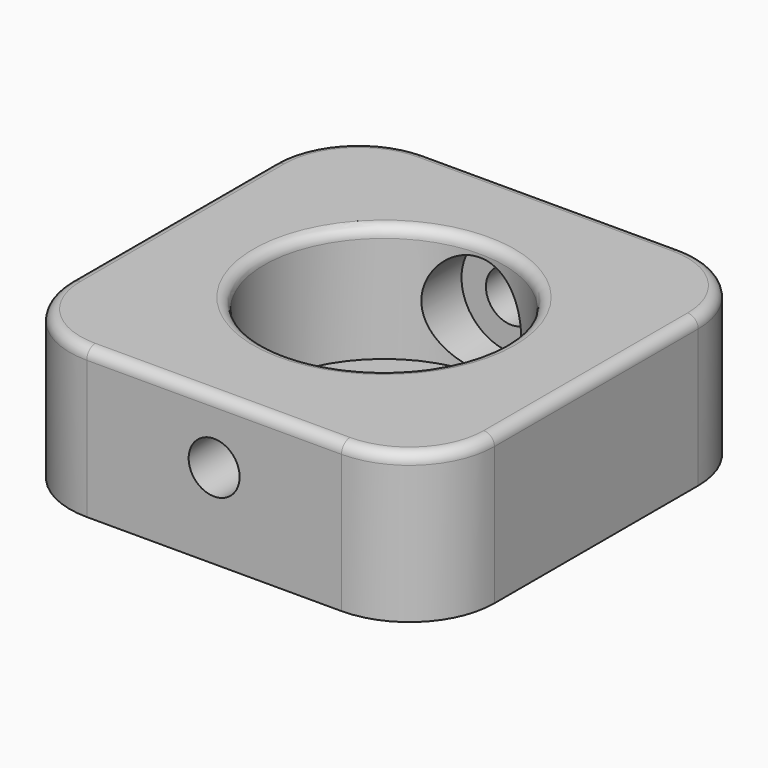
from build123d import *

# Parameters (mm, degrees)
F0_R     = 11.3
F0_R_2   = 8.5
F1_DEPTH = 3
F0_W     = 40
F0_H     = 40
F2_DEPTH = 14
F3_R     = 4.7
F4_DEPTH = 40.001
F5_R     = 4.7
F5_R_2   = 2.4
F6_DEPTH = 5
F7_R     = 4.7
F7_R_2   = 2.4
F8_DEPTH = 5
F9_R     = 8
F10_R    = 1


with BuildPart() as f1:
    # F0 (on Top) → F1 (new body)
    with BuildSketch(Plane.XY):
        Circle(F0_R)
        Circle(F0_R_2, mode=Mode.SUBTRACT)
    extrude(amount=F1_DEPTH)

    # F0 (on Top) → F2 (join)
    with BuildSketch(Plane.XY):
        Rectangle(F0_W, F0_H)
        Circle(F0_R, mode=Mode.SUBTRACT)
    extrude(amount=F2_DEPTH)

    # F3 (on face) → F4 (cut, through all)
    with BuildSketch(Plane.XZ.offset(20)):
        with Locations((0, 8)):
            Circle(F3_R)
    extrude(amount=-F4_DEPTH, mode=Mode.SUBTRACT)

    # F5 (on face) → F6 (join)
    with BuildSketch(Plane.XZ.offset(20)):
        with Locations((0, 8)):
            Circle(F5_R)
        with Locations((0, 8)):
            Circle(F5_R_2, mode=Mode.SUBTRACT)
    extrude(amount=-F6_DEPTH)

    # F7 (on face) → F8 (join)
    with BuildSketch(Plane(origin=(0, 20, 0), x_dir=(-1, 0, 0), z_dir=(0, 1, 0))):
        with Locations((0, 8)):
            Circle(F7_R)
        with Locations((0, 8)):
            Circle(F7_R_2, mode=Mode.SUBTRACT)
    extrude(amount=-F8_DEPTH)

    # F9
    f9_edges = [f1.edges().sort_by_distance(p)[0] for p in [
        (-20, -20, 7),
        (-20, 20, 7),
        (20, -20, 7),
        (20, 20, 7),
    ]]
    fillet(f9_edges, radius=F9_R)

    # F10
    f10_edges = [f1.edges().sort_by_distance(p)[0] for p in [
        (0, -20, 14),
        (-11.3, 0, 14),
    ]]
    fillet(f10_edges, radius=F10_R)


solid = f1.part
